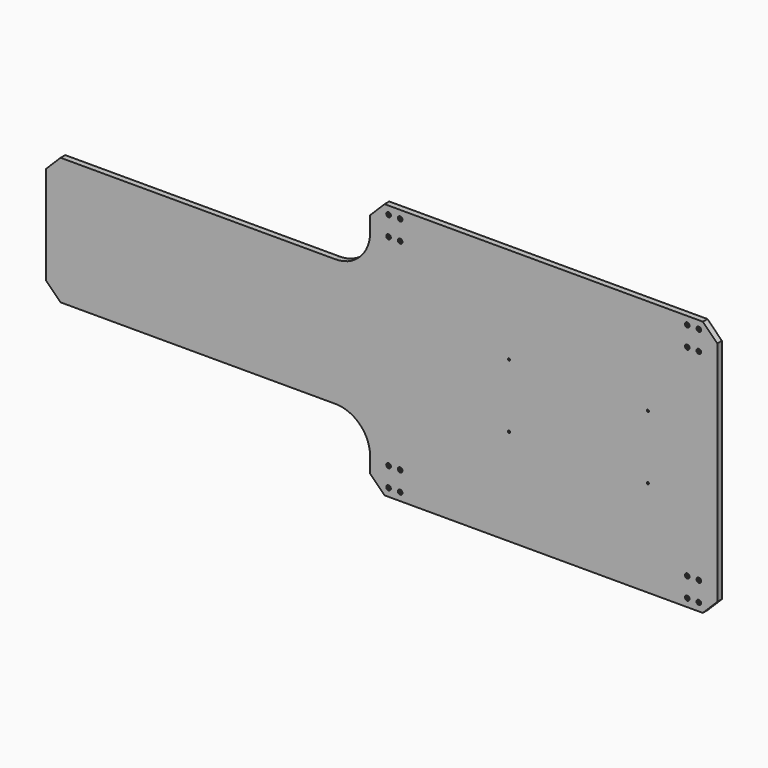
from build123d import *

# Parameters (mm, degrees)
F1_DEPTH       = 12.7
F2_SIZE        = 31.75
F3_R           = 76.2
F5_D           = 4.826
F5_CBORE_D     = 10.16
F5_CBORE_DEPTH = 3.3528
F7_D           = 4.826


# Not quite as in the source:
# - a feature names something its author has since deleted; it is built from what else it names


with BuildPart() as f1:
    # F0 (on Front) → F1 (new body)
    with BuildSketch(Plane.XZ):
        Polygon((381, 139.7), (381, 281.3812), (-381, 281.3812), (-381, 139.7), (-1092.2, 139.7), (-1092.2, 0), (-1092.2, -139.7), (-400.1457989216, -139.7), (-381, -139.7), (-381, -281.3812), (381, -281.3812), (381, -139.7), (381, -69.85), (381, 0), (381, 69.85), align=None)
    extrude(amount=F1_DEPTH)

    # F2
    f2_edges = [f1.edges().sort_by_distance(p)[0] for p in [
        (-381, -6.35, -281.3812),
        (381, -6.35, -281.3812),
        (381, -6.35, 281.3812),
        (-381, -6.35, 281.3812),
        (-1092.2, -6.35, -139.7),
        (-1092.2, -6.35, 139.7),
    ]]
    chamfer(f2_edges, length=F2_SIZE)

    # F3
    f3_edges = [f1.edges().sort_by_distance(p)[0] for p in [
        (-381, -6.35, 139.7),
        (-381, -6.35, -139.7),
    ]]
    fillet(f3_edges, radius=F3_R)

    # F5 (through all)
    with Locations(Plane.XZ.offset(12.7)):
        with Locations((-340.5124, 263.9314), (-315.1124, 263.9314), (-315.1124, 221.0562), (-340.5124, 221.0562), (315.1124, 263.9314), (340.5124, 263.9314), (340.5124, 221.0562), (315.1124, 221.0562), (340.5124, -221.0562), (315.1124, -221.0562), (315.1124, -263.9314), (340.5124, -263.9314), (-315.1124, -221.0562), (-340.5124, -221.0562), (-340.5124, -263.9314), (-315.1124, -263.9314)):
            CounterBoreHole(F5_D / 2, F5_CBORE_D / 2, F5_CBORE_DEPTH)

    # F7 (through all)
    with Locations(Plane.XZ.offset(12.7)):
        with Locations((-76.2, 69.85), (228.6, 69.85), (228.6, -69.85), (-76.2, -69.85)):
            Hole(F7_D / 2)


solid = f1.part
